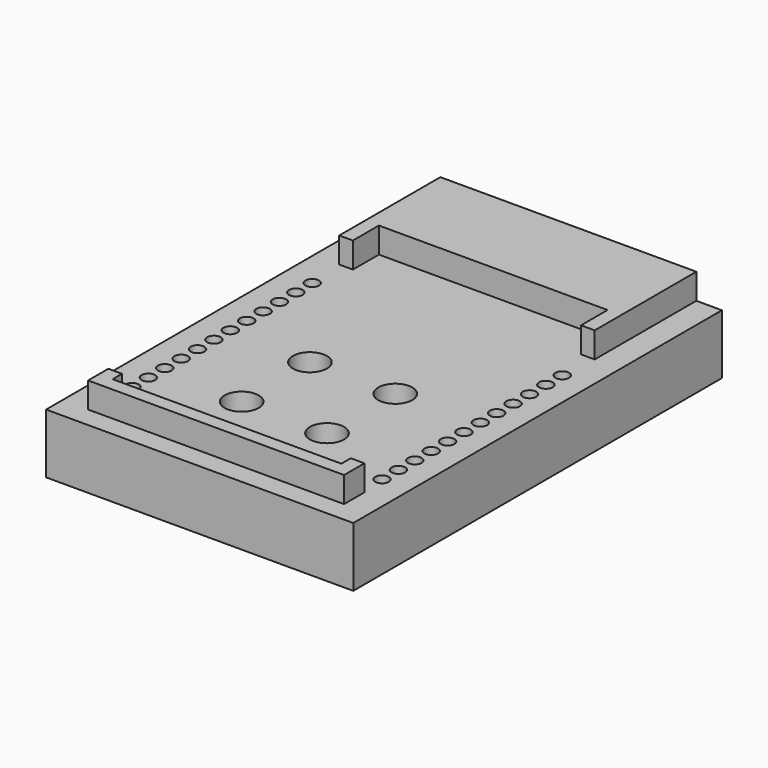
from build123d import *

# Parameters (mm, degrees)
F1_DEPTH = 5
F0_R     = 1
F2_DEPTH = 3.5
F3_R     = 0.4
F4_DEPTH = 12.5


with BuildPart() as f1:
    # F0 (on Top) → F1 (new body)
    with BuildSketch(Plane.XY):
        Polygon((0, 1.4873089967), (0, 0), (15, 0), (15, 1.4873089967), (14.2, 1.4873089967), (14.2, 0.8), (0.8, 0.8), (0.8, 1.4873089967), align=None)
    extrude(amount=F1_DEPTH)

    # F0 (on Top) → F2 (join)
    with BuildSketch(Plane.XY):
        Polygon((0, 18.3973629028), (0, 25.8), (-1.5, 25.8), (-1.5, -1.2), (16.5, -1.2), (16.5, 25.8), (15, 25.8), (15, 18.3544885367), (14.2, 18.3544885367), (14.2, 20.3), (0.8, 20.3), (0.8, 18.3973629028), align=None)
        with Locations((5, 5)):
            Circle(F0_R, mode=Mode.SUBTRACT)
        with Locations((5, 10)):
            Circle(F0_R, mode=Mode.SUBTRACT)
        Polygon((15, 0), (0, 0), (0, 1.4873089967), (0.8, 1.4873089967), (0.8, 0.8), (14.2, 0.8), (14.2, 1.4873089967), (15, 1.4873089967), align=None, mode=Mode.SUBTRACT)
        with Locations((10, 5)):
            Circle(F0_R, mode=Mode.SUBTRACT)
        with Locations((10, 10)):
            Circle(F0_R, mode=Mode.SUBTRACT)
    extrude(amount=F2_DEPTH)

    # F3 (on face) → F4 (cut, symmetric)
    with BuildSketch(Plane.XY.offset(3.5)):
        with Locations((0.175, 3)):
            Circle(F3_R)
        with Locations((0.175, 4.2)):
            Circle(F3_R)
        with Locations((0.175, 5.4)):
            Circle(F3_R)
        with Locations((0.175, 6.6)):
            Circle(F3_R)
        with Locations((0.175, 7.8)):
            Circle(F3_R)
        with Locations((0.175, 9)):
            Circle(F3_R)
        with Locations((0.175, 10.2)):
            Circle(F3_R)
        with Locations((0.175, 11.4)):
            Circle(F3_R)
        with Locations((0.175, 12.6)):
            Circle(F3_R)
        with Locations((0.175, 13.8)):
            Circle(F3_R)
        with Locations((0.175, 15)):
            Circle(F3_R)
        with Locations((0.175, 16.2)):
            Circle(F3_R)
        with Locations((14.825, 3)):
            Circle(F3_R)
        with Locations((14.825, 4.2)):
            Circle(F3_R)
        with Locations((14.825, 5.4)):
            Circle(F3_R)
        with Locations((14.825, 6.6)):
            Circle(F3_R)
        with Locations((14.825, 7.8)):
            Circle(F3_R)
        with Locations((14.825, 9)):
            Circle(F3_R)
        with Locations((14.825, 10.2)):
            Circle(F3_R)
        with Locations((14.825, 11.4)):
            Circle(F3_R)
        with Locations((14.825, 12.6)):
            Circle(F3_R)
        with Locations((14.825, 13.8)):
            Circle(F3_R)
        with Locations((14.825, 15)):
            Circle(F3_R)
        with Locations((14.825, 16.2)):
            Circle(F3_R)
    extrude(amount=F4_DEPTH, both=True, mode=Mode.SUBTRACT)


with BuildPart() as f1b:
    # F0 (on Top) → F1, piece 2 (new body)
    with BuildSketch(Plane.XY):
        Polygon((15, 25.8), (0, 25.8), (0, 18.3973629028), (0.8, 18.3973629028), (0.8, 20.3), (14.2, 20.3), (14.2, 18.3544885367), (15, 18.3544885367), align=None)
    extrude(amount=F1_DEPTH)


solid = Compound([f1.part, f1b.part])
